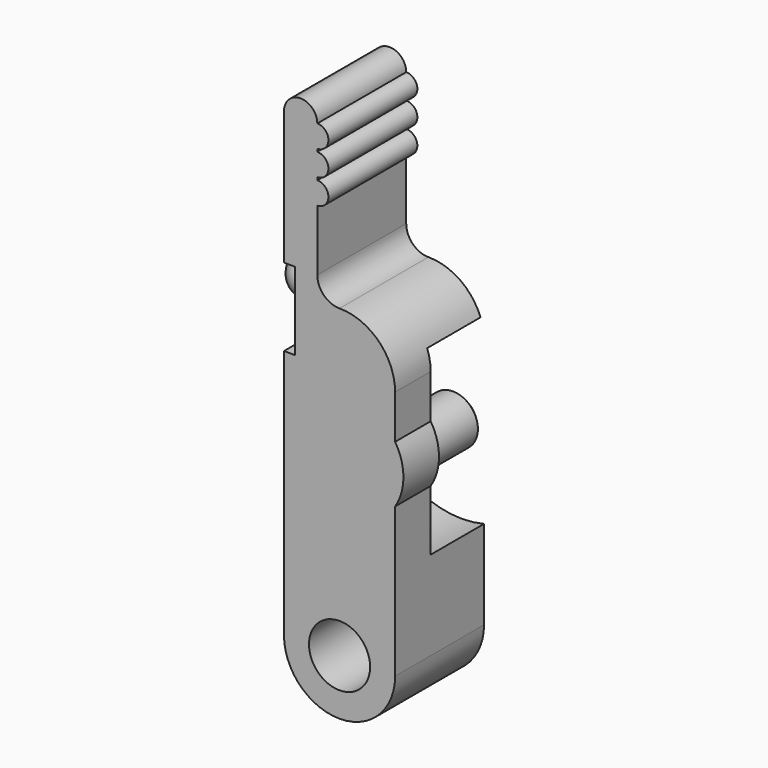
from build123d import *

# Parameters (mm, degrees)
F0_R      = 2.75
F1_DEPTH  = 5
F5_W      = 6
F5_H      = 8.25
F7_DEPTH  = 2.751
F8_R      = 4.99999
F9_R      = 2.25
F10_DEPTH = 5.5
F11_SIZE  = 0.5


# Not quite as in the source:
# - a fillet or chamfer is up to 0.001 mm smaller than in the source, because OpenCascade refuses the exact size


with BuildPart() as f1:
    # F0 (on Front) → F1 (new body, symmetric)
    with BuildSketch(Plane.XZ):
        with BuildLine():
            ThreePointArc((-2, 41.5), (-3.5, 43), (-5, 41.5))
            Line((-5, 41.5), (-5, 29.5))
            Line((-5, 29.5), (-4, 29.5))
            Line((-4, 29.5), (-4, 22.5))
            Line((-4, 22.5), (-5, 22.5))
            Line((-5, 22.5), (-5, 0))
            ThreePointArc((-5, 0), (0, -5), (5, 0))
            Line((5, 0), (5, 13.4382623085))
            ThreePointArc((5, 13.4382623085), (5.75, 16), (5, 18.5617376915))
            Line((5, 18.5617376915), (5, 27.5))
            Line((5, 27.5), (0, 27.5))
            ThreePointArc((0, 27.5), (-1.4142135624, 28.0857864376), (-2, 29.5))
            Line((-2, 29.5), (-2, 35))
            Line((-2, 35), (-2, 37))
            Line((-2, 37), (-2, 37.25))
            Line((-2, 37.25), (-2, 39.25))
            Line((-2, 39.25), (-2, 39.5))
            Line((-2, 39.5), (-2, 41.5))
        make_face()
        Circle(F0_R, mode=Mode.SUBTRACT)
        with BuildLine():
            ThreePointArc((-2, 39.5), (-1, 40.5), (-2, 41.5))
            Line((-2, 41.5), (-2, 39.5))
        make_face()
        with BuildLine():
            ThreePointArc((-2, 37.25), (-1, 38.25), (-2, 39.25))
            Line((-2, 39.25), (-2, 37.25))
        make_face()
        with BuildLine():
            ThreePointArc((-2, 35), (-1, 36), (-2, 37))
            Line((-2, 37), (-2, 35))
        make_face()
    extrude(amount=F1_DEPTH, both=True)

    # F2 (on Front) → F3 (revolve)
    with BuildSketch(Plane.XZ):
        with BuildLine():
            Line((-3.3124492232, 25.9398471014), (-3.1381377377, 27.9322364976))
            Line((-3.1381377377, 27.9322364976), (-6.126721832, 28.1937037259))
            ThreePointArc((-6.126721832, 28.1937037259), (-7.5866085368, 27.7334032159), (-8.2934227136, 26.3756258152))
            Line((-8.2934227136, 26.3756258152), (-3.3124492232, 25.9398471014))
        make_face()
    revolve(axis=Axis((-3.9560072501, 0, 25.9961511331), (-0.9961946981, 0, 0.0871557427)))

    # F5 (on offset) → F6 (revolve, cut)
    with BuildSketch(Plane.YZ.offset(3)):
        with Locations((2, 20.125)):
            Rectangle(F5_W, F5_H)
    revolve(axis=Axis((3, 0.0511605343, 16), (0, 1, 0)), mode=Mode.SUBTRACT)

    # F5 (on offset) → F7 (cut, through all)
    with BuildSketch(Plane.YZ.offset(3)):
        with Locations((2, 20.125)):
            Rectangle(F5_W, F5_H)
    extrude(amount=F7_DEPTH, mode=Mode.SUBTRACT)

    # F8 (radius 5 in the source; OpenCascade refuses exactly that, so slightly less here)
    f8_edges = [f1.edges().sort_by_distance(p)[0] for p in [
        (5, 0, 27.5),
    ]]
    fillet(f8_edges, radius=F8_R)

    # F9 (on face) → F10 (join)
    with BuildSketch(Plane(origin=(0, -1, 0), x_dir=(-1, 0, 0), z_dir=(0, 1, 0))):
        with Locations((-3, 16)):
            Circle(F9_R)
    extrude(amount=F10_DEPTH)

    # F11
    f11_edges = [f1.edges().sort_by_distance(p)[0] for p in [
        (5.25, 4.5, 16),
    ]]
    chamfer(f11_edges, length=F11_SIZE)


solid = f1.part
